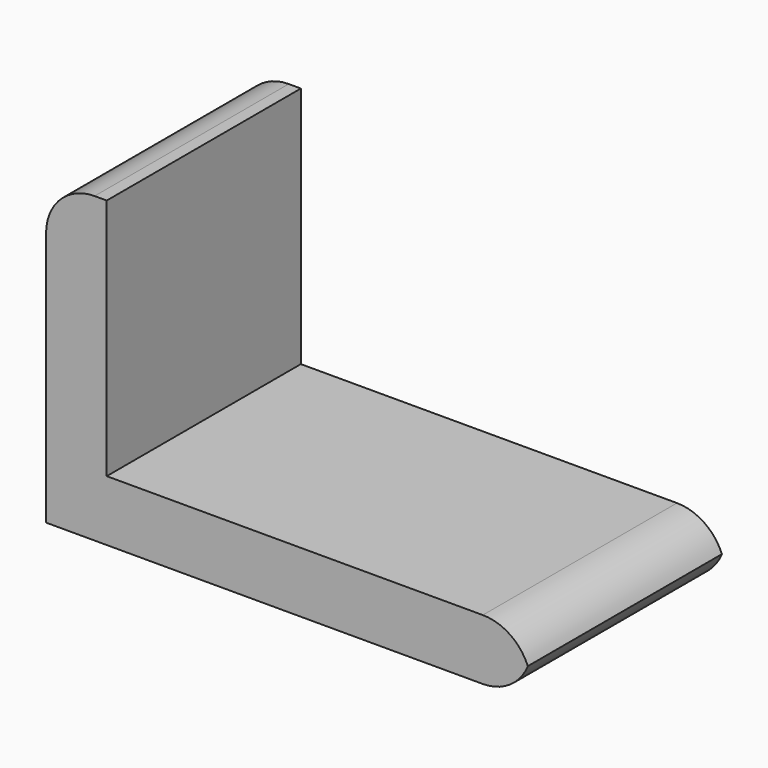
from build123d import *

# Parameters (mm, degrees)
F1_DEPTH    = 25.4
F2_T1_DEPTH = 50.8
F3_R        = 5.08


# Not quite as in the source:
# - a fillet or chamfer that OpenCascade refuses, or shapes differently, is made with other operations: its cross-section is extruded or revolved along the edge and cut away or added


with BuildPart() as f1:
    # F0 (on Front) → F1 (new body)
    with BuildSketch(Plane.XZ):
        Polygon((0, 31.75), (0, 0), (50.8, 0), (50.8, 6.35), (6.35, 6.35), (6.35, 31.75), align=None)
    extrude(amount=-F1_DEPTH)

    # F2: fillet of radius 5.08 on 2 edges, made by hand

    # F2_s2 → F2_t1 (cut)
    with BuildSketch(Plane.XZ.offset(-38.1)):
        with BuildLine():
            ThreePointArc((50.8, 1.27), (49.3121024484, 4.8621024484), (45.72, 6.35))
            Line((45.72, 6.35), (50.8, 6.35))
            Line((50.8, 6.35), (50.8, 1.27))
        make_face()
        with BuildLine():
            ThreePointArc((45.72, 0), (49.3121024484, 1.4878975516), (50.8, 5.08))
            Line((50.8, 5.08), (50.8, 0))
            Line((50.8, 0), (45.72, 0))
        make_face()
    extrude(amount=F2_T1_DEPTH, mode=Mode.SUBTRACT)

    # F3
    f3_edges = [f1.edges().sort_by_distance(p)[0] for p in [
        (0, 12.7, 31.75),
    ]]
    fillet(f3_edges, radius=F3_R)


solid = f1.part
